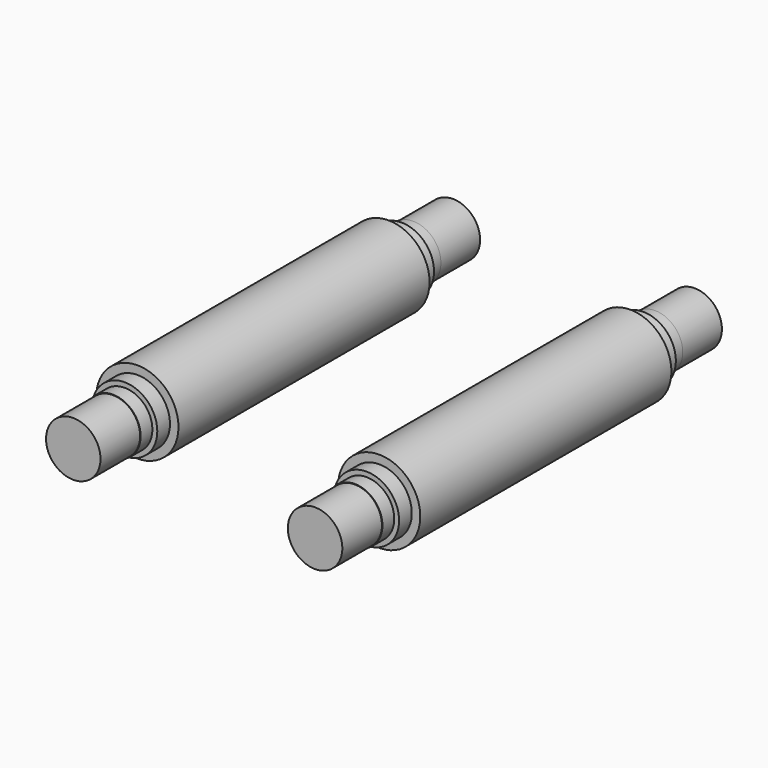
from build123d import *

# Parameters (mm, degrees)
F0_R      = 8.5
F1_DEPTH  = 32.445
F2_R      = 6.74
F3_DEPTH  = 3.28
F4_R      = 5.73
F5_DEPTH  = 3.04
F6_R      = 5.63
F7_DEPTH  = 10.25
F8_R      = 6.74
F9_DEPTH  = 3.36
F10_R     = 5.73
F11_DEPTH = 3.04
F12_R     = 5.63
F13_DEPTH = 10.25


with BuildPart() as f1:
    # F0 (on Front) → F1 (new body, symmetric)
    with BuildSketch(Plane.XZ):
        Circle(F0_R)
    extrude(amount=F1_DEPTH, both=True)

    # F2 (on face) → F3 (join)
    with BuildSketch(Plane.XZ.offset(32.445)):
        Circle(F2_R)
    extrude(amount=F3_DEPTH)

    # F4 (on face) → F5 (join)
    with BuildSketch(Plane.XZ.offset(35.725)):
        Circle(F4_R)
    extrude(amount=F5_DEPTH)

    # F6 (on face) → F7 (join)
    with BuildSketch(Plane.XZ.offset(38.765)):
        Circle(F6_R)
    extrude(amount=F7_DEPTH)

    # F8 (on face) → F9 (join)
    with BuildSketch(Plane(origin=(0, 32.445, 0), x_dir=(-1, 0, 0), z_dir=(0, 1, 0))):
        Circle(F8_R)
    extrude(amount=F9_DEPTH)

    # F10 (on face) → F11 (join)
    with BuildSketch(Plane(origin=(0, 35.805, 0), x_dir=(-1, 0, 0), z_dir=(0, 1, 0))):
        Circle(F10_R)
    extrude(amount=F11_DEPTH)

    # F12 (on face) → F13 (join)
    with BuildSketch(Plane(origin=(0, 38.845, 0), x_dir=(-1, 0, 0), z_dir=(0, 1, 0))):
        Circle(F12_R)
    extrude(amount=F13_DEPTH)


with BuildPart() as f15_1:
    # F15: instance of F1
    add(f1.part.mirror(Plane.YZ.offset(25)))


solid = Compound([f1.part, f15_1.part])
